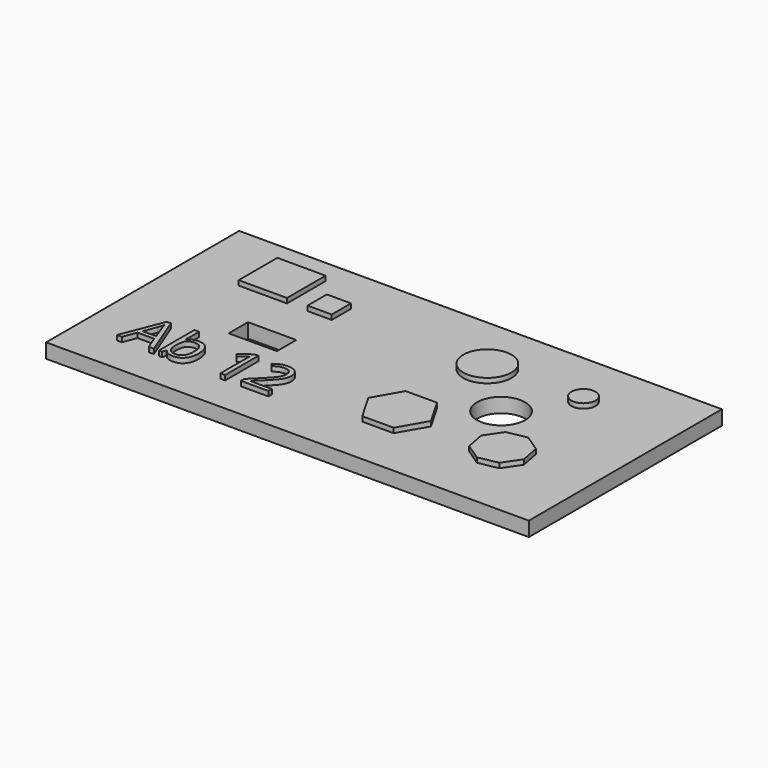
from build123d import *

# Parameters (mm, degrees)
F0_W           = 200
F0_H           = 100
F1_DEPTH       = 6
F2_W           = 20
F2_H           = 20
F3_DEPTH       = 2
F2_W_2         = 10
F2_H_2         = 10
F4_DEPTH       = 2
F2_R           = 10
F5_DEPTH       = 2
F2_R_2         = 5
F6_DEPTH       = 2
F7_DEPTH       = 2
F8_DEPTH       = 2
F9_TEXT_SIZE   = 24.1791312065
F10_DEPTH      = 2
F11_W          = 20
F11_H          = 10
F12_DEPTH      = 25
F11_R          = 10
F13_DEPTH      = 25
F13_DEPTH_BACK = 25


# Not quite as in the source:
# - Text() gives the source's letters only with a copy of the font that has no kerning and outlines rounded to 1/6400 em; it was checked with that copy


with BuildPart() as f1:
    # F0 (on Top) → F1 (new body)
    with BuildSketch(Plane.XY):
        Rectangle(F0_W, F0_H)
    extrude(amount=F1_DEPTH)

    # F2 (on face) → F3 (join)
    with BuildSketch(Plane.XY.offset(6)):
        with Locations((-66.1655226614, 29.9572380581)):
            Rectangle(F2_W, F2_H)
    extrude(amount=F3_DEPTH)

    # F2 (on face) → F4 (join)
    with BuildSketch(Plane.XY.offset(6)):
        with Locations((-42.6340532938, 24.9572380581)):
            Rectangle(F2_W_2, F2_H_2)
    extrude(amount=F4_DEPTH)

    # F2 (on face) → F5 (join)
    with BuildSketch(Plane.XY.offset(6)):
        with Locations((23.1996364892, 24.5436728001)):
            Circle(F2_R)
    extrude(amount=F5_DEPTH)

    # F2 (on face) → F6 (join)
    with BuildSketch(Plane.XY.offset(6)):
        with Locations((61.7041923106, 26.1821653694)):
            Circle(F2_R_2)
    extrude(amount=F6_DEPTH)

    # F2 (on face) → F7 (join)
    with BuildSketch(Plane.XY.offset(6)):
        Polygon((27.5815651832, -29.4612292871), (34.050144154, -18.2115267292), (27.5419054393, -6.9847217352), (14.5650877537, -7.007619299), (8.0965087829, -18.2573218569), (14.6047474977, -29.4841268509), align=None)
    extrude(amount=F7_DEPTH)

    # F2 (on face) → F8 (join)
    with BuildSketch(Plane.XY.offset(6)):
        Polygon((69.657634835, -27.2665422236), (74.2984452441, -20.4062137927), (72.729009, -12.2736805275), (65.868680569, -7.6328701183), (57.7361473039, -9.2023063625), (53.0953368947, -16.0626347934), (54.6647731389, -24.1951680586), (61.5251015698, -28.8359784677), align=None)
    extrude(amount=F8_DEPTH)

    # F9 (on face) → F10 (join)
    with BuildSketch(Plane.XY.offset(6)):
        with Locations((-82.9207524657, -34.6783101559)):
            Text('Ab 12', F9_TEXT_SIZE, font='Open Sans', text_align=(TextAlign.LEFT, TextAlign.BOTTOM))
    extrude(amount=F10_DEPTH)

    # F11 (on face) → F12 (cut)
    with BuildSketch(Plane.XY.offset(6)):
        with Locations((-47.8234738111, -3.1584628208)):
            Rectangle(F11_W, F11_H)
    extrude(amount=-F12_DEPTH, mode=Mode.SUBTRACT)

    # F11 (on face) → F13 (cut, two sides)
    with BuildSketch(Plane.XY.offset(6)) as f13_sk:
        with Locations((45.0585149229, 4.3010399677)):
            Circle(F11_R)
    extrude(amount=-F13_DEPTH, mode=Mode.SUBTRACT)
    extrude(f13_sk.sketch, amount=F13_DEPTH_BACK, mode=Mode.SUBTRACT)


solid = f1.part
